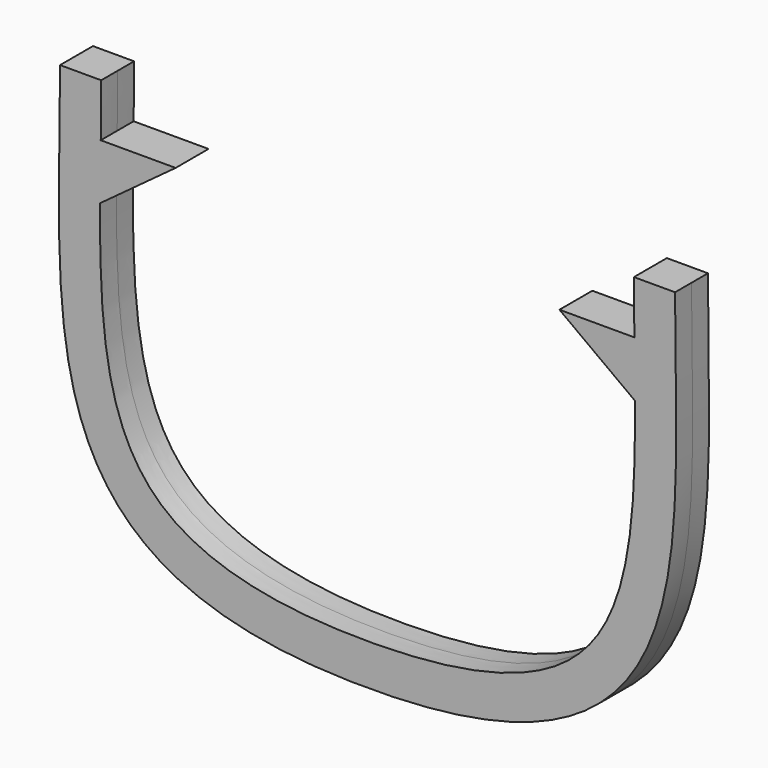
from build123d import *

# Parameters (mm, degrees)
F1_DEPTH = 5


# Not quite as in the source:
# - ends of sketch curves that miss each other by under 0.0002 mm in the source are joined
# - the dataset's text gives a spline's control points without its knots; the knots are read off the source's solid


with BuildPart() as f1:
    # F0 (on Front) → F1 (new body, symmetric)
    with BuildSketch(Plane.XZ):
        with BuildLine():
            add(Edge.make_bspline(
                [(0, 0), (-83.6641341448, 0), (-74.7610164563, 50.3125078976), (-74.7610164563, 109)],
                knots=[0, 0, 0, 0, 132.1749203956, 132.1749203956, 132.1749203956, 132.1749203956], degree=3))
            add(Edge.make_bspline(
                [(0, 0), (83.6641341448, 0), (74.7610164563, 50.3125078976), (74.7610164563, 109)],
                knots=[0, 0, 0, 0, 132.1749203956, 132.1749203956, 132.1749203956, 132.1749203956], degree=3))
            Line((74.7610164563, 109), (64.7610164563, 109))
            add(Edge.make_bspline(
                [(64.8651773016, 96.1271052425), (64.809283505, 100.3316929307), (64.7610087024, 104.6288918899), (64.7610164563, 109)],
                knots=[0.9267807006, 0.9267807006, 0.9267807006, 0.9267807006, 1, 1, 1, 1], degree=3))
            add(Edge.make_bspline(
                [(65.0234491439, 82.6084248881), (65.0139858714, 84.1724141651), (64.9721404166, 88.5989382646), (64.9047054038, 93.153620136), (64.8651773016, 96.1271052425)],
                knots=[0.8462097598, 0.8462097598, 0.8462097598, 0.8462097598, 0.875, 0.9267807006, 0.9267807006, 0.9267807006, 0.9267807006], degree=3))
            add(Edge.make_bspline(
                [(0, 10), (4.9784405013, 10), (14.1558453385, 10.3748520854), (25.6971414705, 11.9511255345), (35.1427822184, 14.4036535664), (42.6707713147, 17.5717741572), (48.5489406763, 21.3119415285), (53.1312678675, 25.5800594028), (56.7549643638, 30.4771390793), (59.6251039368, 36.1647439539), (61.8230057051, 42.7389566362), (63.3915232472, 50.196336895), (64.3908810398, 58.469845885), (65.0061181592, 69.0869180815), (65.0550730263, 77.3819650971), (65.0234491439, 82.6084248881)],
                knots=[0, 0, 0, 0, 0.0625, 0.125, 0.1875, 0.25, 0.3125, 0.375, 0.4375, 0.5, 0.5625, 0.625, 0.6875, 0.75, 0.8462097598, 0.8462097598, 0.8462097598, 0.8462097598], degree=3))
            add(Edge.make_bspline(
                [(0, 10), (-4.9784405013, 10), (-14.1558453385, 10.3748520854), (-25.6971414705, 11.9511255345), (-35.1427822184, 14.4036535664), (-42.6707713147, 17.5717741572), (-48.5489406763, 21.3119415285), (-53.1312678675, 25.5800594028), (-56.7549643638, 30.4771390793), (-59.6251039368, 36.1647439539), (-61.8230057051, 42.7389566362), (-63.3915232472, 50.196336895), (-64.3908810398, 58.469845885), (-65.0061181601, 69.0869180966), (-65.0550730265, 77.3819651301), (-65.0234491436, 82.6084249395)],
                knots=[0, 0, 0, 0, 0.0625, 0.125, 0.1875, 0.25, 0.3125, 0.375, 0.4375, 0.5, 0.5625, 0.625, 0.6875, 0.75, 0.8462097601, 0.8462097601, 0.8462097601, 0.8462097601], degree=3))
            add(Edge.make_bspline(
                [(-65.0234491436, 82.6084249395), (-65.0139858711, 84.1724141997), (-64.9721404166, 88.5989382611), (-64.9047054044, 93.1536200922), (-64.8651773025, 96.1271051757)],
                knots=[0.8462097601, 0.8462097601, 0.8462097601, 0.8462097601, 0.875, 0.9267807002, 0.9267807002, 0.9267807002, 0.9267807002], degree=3))
            add(Edge.make_bspline(
                [(-64.8651773025, 96.1271051757), (-64.8092835055, 100.3316928852), (-64.7610087024, 104.6288918667), (-64.7610087024, 109)],
                knots=[0.9267807002, 0.9267807002, 0.9267807002, 0.9267807002, 1, 1, 1, 1], degree=3))
            Line((-64.7610087024, 109), (-74.7610164563, 109))
        make_face()
        with BuildLine():
            add(Edge.make_bspline(
                [(65.0234491439, 82.6084248881), (65.0139858714, 84.1724141651), (64.9721404166, 88.5989382646), (64.9047054038, 93.153620136), (64.8651773016, 96.1271052425)],
                knots=[0.8462097598, 0.8462097598, 0.8462097598, 0.8462097598, 0.875, 0.9267807006, 0.9267807006, 0.9267807006, 0.9267807006], degree=3))
            Line((64.8651773016, 96.1271052425), (46.6552594428, 96.1271063344))
            Line((46.6552594428, 96.1271063344), (65.0234491439, 82.6084248881))
        make_face()
        with BuildLine():
            Line((-46.6585347408, 96.1271062676), (-64.8652594437, 96.1271062676))
            add(Edge.make_bspline(
                [(-65.0234491436, 82.6084249395), (-65.0139858711, 84.1724141997), (-64.9721404166, 88.5989382611), (-64.9047054044, 93.1536200922), (-64.8652594437, 96.1271062676)],
                knots=[0.8462097601, 0.8462097601, 0.8462097601, 0.8462097601, 0.875, 0.9267807002, 0.9267807002, 0.9267807002, 0.9267807002], degree=3))
            Line((-65.0234491436, 82.6084249395), (-46.6585347408, 96.1271062676))
        make_face()
    extrude(amount=F1_DEPTH, both=True)


solid = f1.part
